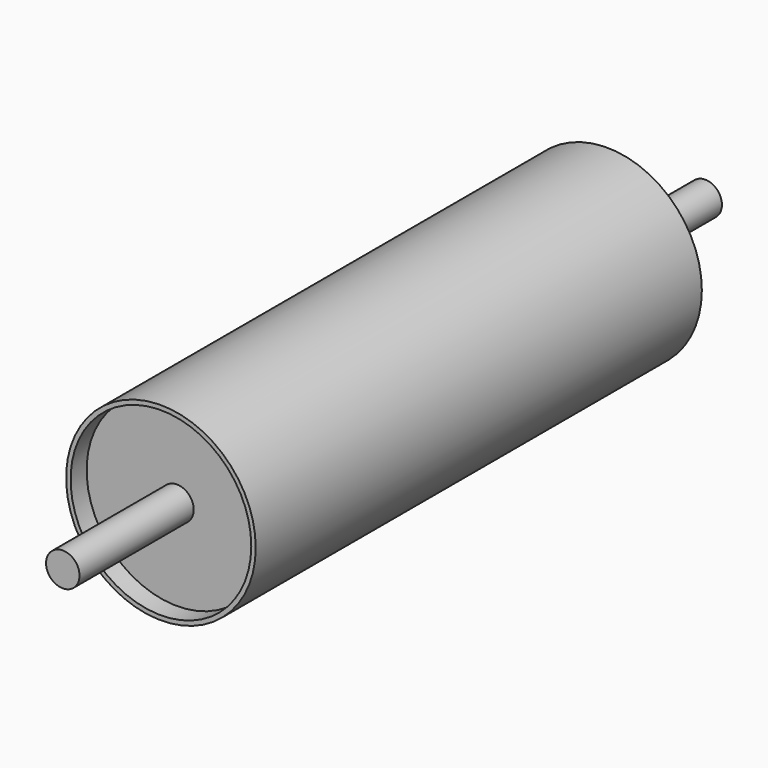
from build123d import *

# Parameters (mm, degrees)
F0_R           = 15
F1_DEPTH       = 360
F1_DEPTH_BACK  = 360
F2_R           = 85
F3_DEPTH       = 250
F3_DEPTH_BACK  = 250
F4_R           = 81
F5_DEPTH       = 610.001
F7_R           = 81
F8_DEPTH       = 2
F8_DEPTH_BACK  = 2
F9_R           = 15
F10_DEPTH      = 4
F10_DEPTH_BACK = 4
F12_R          = 81
F13_DEPTH      = 2
F13_DEPTH_BACK = 2
F14_R          = 15
F15_DEPTH      = 25
F15_DEPTH_BACK = 25


with BuildPart() as f1:
    # F0 (on Front) → F1 (new body, two sides)
    with BuildSketch(Plane.XZ) as f1_sk:
        Circle(F0_R)
    extrude(amount=F1_DEPTH)
    extrude(f1_sk.sketch, amount=-F1_DEPTH_BACK)


with BuildPart() as f3:
    # F2 (on Front) → F3 (new body, two sides)
    with BuildSketch(Plane.XZ) as f3_sk:
        Circle(F2_R)
    extrude(amount=F3_DEPTH)
    extrude(f3_sk.sketch, amount=-F3_DEPTH_BACK)

    # F4 (on face) → F5 (cut, through all)
    with BuildSketch(Plane.XZ.offset(250)):
        Circle(F4_R)
    extrude(amount=-F5_DEPTH, mode=Mode.SUBTRACT)

    # F7 (on offset) → F8 (join, two sides)
    with BuildSketch(Plane.XZ.offset(230)) as f8_sk:
        Circle(F7_R)
    extrude(amount=F8_DEPTH)
    extrude(f8_sk.sketch, amount=-F8_DEPTH_BACK)

    # F9 (on offset) → F10 (cut, two sides)
    with BuildSketch(Plane.XZ.offset(230)) as f10_sk:
        Circle(F9_R)
    extrude(amount=-F10_DEPTH, mode=Mode.SUBTRACT)
    extrude(f10_sk.sketch, amount=F10_DEPTH_BACK, mode=Mode.SUBTRACT)

    # F12 (on offset) → F13 (join, two sides)
    with BuildSketch(Plane(origin=(0, 230, 0), x_dir=(-1, 0, 0), z_dir=(0, 1, 0))) as f13_sk:
        Circle(F12_R)
    extrude(amount=F13_DEPTH)
    extrude(f13_sk.sketch, amount=-F13_DEPTH_BACK)

    # F14 (on offset) → F15 (cut, two sides)
    with BuildSketch(Plane(origin=(0, 230, 0), x_dir=(-1, 0, 0), z_dir=(0, 1, 0))) as f15_sk:
        Circle(F14_R)
    extrude(amount=F15_DEPTH, mode=Mode.SUBTRACT)
    extrude(f15_sk.sketch, amount=-F15_DEPTH_BACK, mode=Mode.SUBTRACT)


solid = Compound([f1.part, f3.part])
